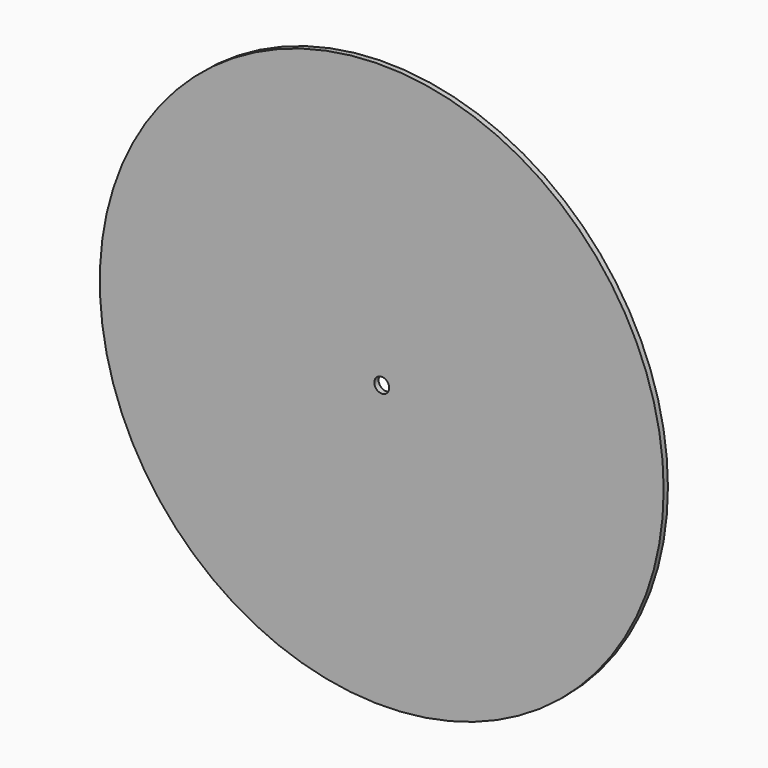
from build123d import *

# Parameters (mm, degrees)
F0_R     = 60.325
F0_R_2   = 1.5875
F1_DEPTH = 1.143


# Not quite as in the source:
# - a feature names something its author has since deleted; it is built from what else it names


with BuildPart() as f1:
    # F0 (on Front) → F1 (new body)
    with BuildSketch(Plane.XZ):
        Circle(F0_R)
        Circle(F0_R_2, mode=Mode.SUBTRACT)
    extrude(amount=F1_DEPTH)


solid = f1.part
